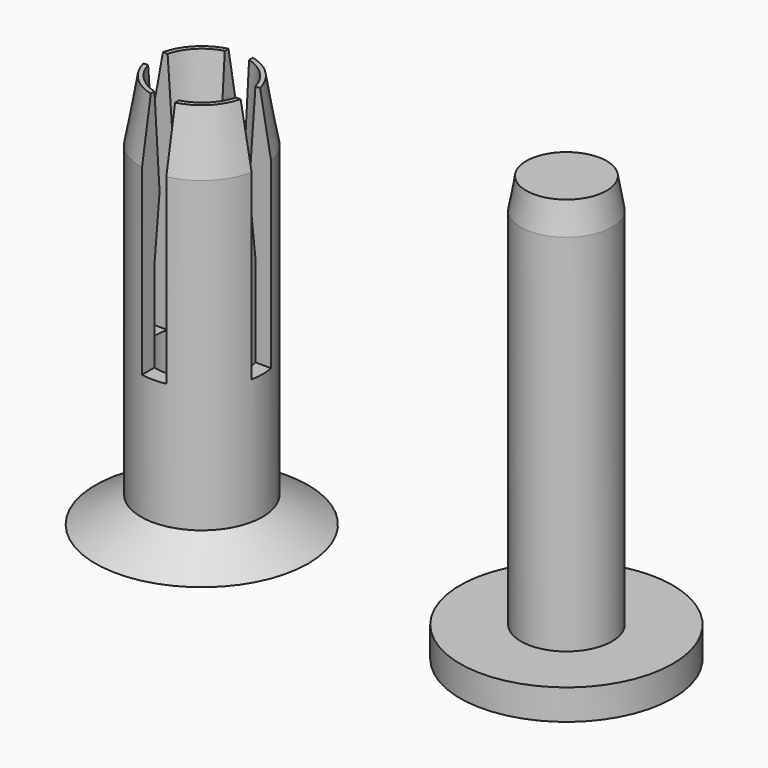
from build123d import *

# Parameters (mm, degrees)
F0_R      = 3.5
F1_DEPTH  = 1
F2_SIZE2  = 1.732041
F2_SIZE   = 0.99999
F3_R      = 2
F4_DEPTH  = 13
F5_SIZE2  = 0.3526539614
F5_SIZE   = 2
F8_R      = 1.5
F9_DEPTH  = 13
F10_SIZE2 = 0.1763269807
F10_SIZE  = 1
F11_W     = 2.1
F11_H     = 0.8
F11_W_2   = 0.8
F11_H_2   = 2.1
F12_DEPTH = 8


# Not quite as in the source:
# - a fillet or chamfer is up to 0.001 mm smaller than in the source, because OpenCascade refuses the exact size


with BuildPart() as f1:
    # F0 (on Top) → F1 (new body)
    with BuildSketch(Plane.XY):
        with Locations((-6, 0)):
            Circle(F0_R)
    extrude(amount=F1_DEPTH)

    # F2 (size 1 and 1.7320508076 in the source; OpenCascade refuses exactly that, so slightly less here)
    f2_edges = [f1.edges().sort_by_distance(p)[0] for p in [
        (-9.5, 0, 1),
    ]]
    f2_side = f1.faces().sort_by_distance((-9.5, 0, 0.5))[0]
    chamfer(f2_edges, length=F2_SIZE, length2=F2_SIZE2, reference=f2_side)

    # F3 (on Top) → F4 (join)
    with BuildSketch(Plane.XY):
        with Locations((-6, 0)):
            Circle(F3_R)
    extrude(amount=F4_DEPTH)

    # F5
    f5_edges = [f1.edges().sort_by_distance(p)[0] for p in [
        (-8, 0, 13),
    ]]
    f5_side = f1.faces().sort_by_distance((-8, 0, 6.933016))[0]
    chamfer(f5_edges, length=F5_SIZE, length2=F5_SIZE2, reference=f5_side)

    # F6 (on Front) → F7 (revolve, cut)
    with BuildSketch(Plane.XZ):
        Polygon((-4.5, 13), (-6, 13), (-6, 0), (-4.5, 0), (-4.5, 8), (-4.7, 10), align=None)
    revolve(axis=Axis((-6, 0, 6.5), (0, 0, -1)), mode=Mode.SUBTRACT)

    # F11 (on face) → F12 (cut)
    with BuildSketch(Plane.XY.offset(13)):
        with Locations((-7.45, 0)):
            Rectangle(F11_W, F11_H)
        with Locations((-6, 1.45)):
            Rectangle(F11_W_2, F11_H_2)
        with Locations((-6, 0)):
            Rectangle(F11_W_2, F11_H)
        with Locations((-4.55, 0)):
            Rectangle(F11_W, F11_H)
        with Locations((-6, -1.45)):
            Rectangle(F11_W_2, F11_H_2)
    extrude(amount=-F12_DEPTH, mode=Mode.SUBTRACT)


with BuildPart() as f1b:
    # F0 (on Top) → F1, piece 2 (new body)
    with BuildSketch(Plane.XY):
        with Locations((6, 0)):
            Circle(F0_R)
    extrude(amount=F1_DEPTH)

    # F8 (on face) → F9 (join)
    with BuildSketch(Plane.XY.offset(1)):
        with Locations((6, 0)):
            Circle(F8_R)
    extrude(amount=F9_DEPTH)

    # F10
    f10_edges = [f1b.edges().sort_by_distance(p)[0] for p in [
        (4.5, 0, 14),
    ]]
    f10_side = f1b.faces().sort_by_distance((4.5, 0, 7.5))[0]
    chamfer(f10_edges, length=F10_SIZE, length2=F10_SIZE2, reference=f10_side)


solid = Compound([f1.part, f1b.part])
